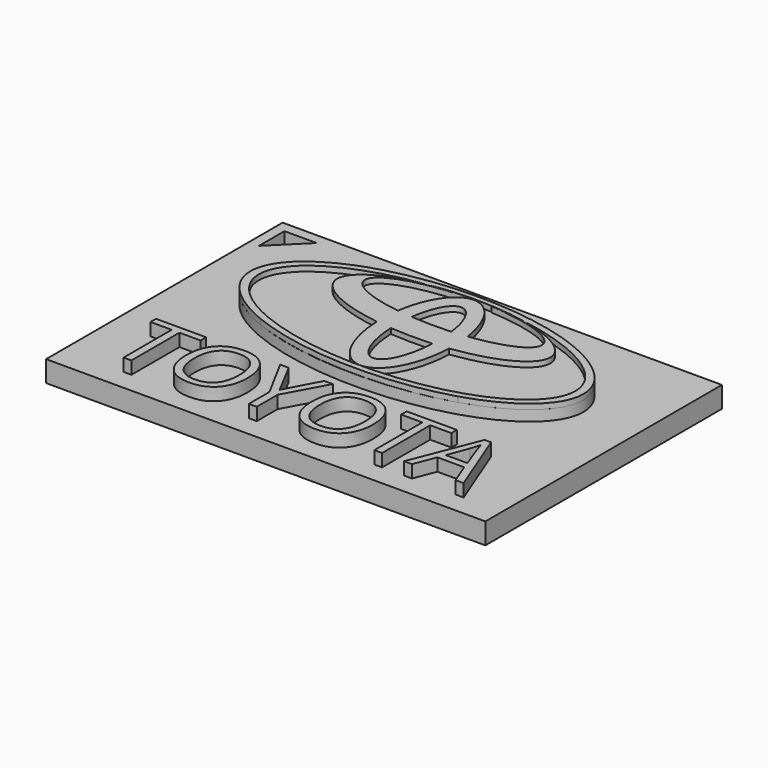
from build123d import *

# Parameters (mm, degrees)
F0_W         = 66.04
F0_H         = 44.45
F0_TEXT_SIZE = 14.1111111111
F1_DEPTH     = 3.175
F2_DEPTH     = 1.5875
F4_DEPTH     = 1.905
F6_DEPTH     = 0.79375


# Not quite as in the source:
# - a feature names something its author has since deleted; it is built from what else it names
# - Text() gives the source's letters only with a copy of the font that has no kerning and outlines rounded to 1/6400 em; it was checked with that copy


with BuildPart() as f1:
    # F0 (on Top) → F1 (new body)
    with BuildSketch(Plane.XY):
        with Locations((3.48807069, -6.6769314361)):
            Rectangle(F0_W, F0_H)
        Polygon((-19.2232334766, -16.7264181777), (-19.2232334766, -25.7597341499), (-20.3940147266, -25.7597341499), (-20.3940147266, -16.7264181777), (-23.5844487544, -16.7264181777), (-23.5844487544, -15.6857237332), (-16.0327994489, -15.6857237332), (-16.0327994489, -16.7264181777), align=None, mode=Mode.SUBTRACT)
        with BuildLine():
            add(Edge.make_bspline(
                [(-6.9906640322, -16.9050119277), (-5.7713758378, -18.2830501221), (-5.7713758378, -20.7083973443)],
                knots=[0, 0, 0, 1, 1, 1], degree=2))
            add(Edge.make_bspline(
                [(-5.7713758378, -20.7083973443), (-5.7713758378, -23.1271299832), (-6.9950737544, -24.5128851915)],
                knots=[0, 0, 0, 1, 1, 1], degree=2))
            add(Edge.make_bspline(
                [(-6.9950737544, -24.5128851915), (-8.2187716711, -25.8986403999), (-10.3949695878, -25.8986403999)],
                knots=[0, 0, 0, 1, 1, 1], degree=2))
            add(Edge.make_bspline(
                [(-10.3949695878, -25.8986403999), (-12.6196744489, -25.8986403999), (-13.8290407683, -24.5371386638)],
                knots=[0, 0, 0, 1, 1, 1], degree=2))
            add(Edge.make_bspline(
                [(-13.8290407683, -24.5371386638), (-15.0384070878, -23.1756369277), (-15.0384070878, -20.6951681777)],
                knots=[0, 0, 0, 1, 1, 1], degree=2))
            add(Edge.make_bspline(
                [(-15.0384070878, -20.6951681777), (-15.0384070878, -18.2345431777), (-13.8257334766, -16.8807584554)],
                knots=[0, 0, 0, 1, 1, 1], degree=2))
            add(Edge.make_bspline(
                [(-13.8257334766, -16.8807584554), (-12.6130598655, -15.5269737332), (-10.3817404211, -15.5269737332)],
                knots=[0, 0, 0, 1, 1, 1], degree=2))
            add(Edge.make_bspline(
                [(-10.3817404211, -15.5269737332), (-8.2099522266, -15.5269737332), (-6.9906640322, -16.9050119277)],
                knots=[0, 0, 0, 1, 1, 1], degree=2))
        make_face(mode=Mode.SUBTRACT)
        Polygon((-3.6304556989, -15.6857237332), (-0.9625737544, -20.7238313721), (1.7229470789, -15.6857237332), (2.9907422178, -15.6857237332), (-0.3716709766, -21.852720261), (-0.3716709766, -25.7597341499), (-1.5556813933, -25.7597341499), (-1.5556813933, -21.9078417888), (-4.9114800044, -15.6857237332), align=None, mode=Mode.SUBTRACT)
        with BuildLine():
            add(Edge.make_bspline(
                [(11.9005859678, -16.9050119277), (13.1198741622, -18.2830501221), (13.1198741622, -20.7083973443)],
                knots=[0, 0, 0, 1, 1, 1], degree=2))
            add(Edge.make_bspline(
                [(13.1198741622, -20.7083973443), (13.1198741622, -23.1271299832), (11.8961762456, -24.5128851915)],
                knots=[0, 0, 0, 1, 1, 1], degree=2))
            add(Edge.make_bspline(
                [(11.8961762456, -24.5128851915), (10.6724783289, -25.8986403999), (8.4962804122, -25.8986403999)],
                knots=[0, 0, 0, 1, 1, 1], degree=2))
            add(Edge.make_bspline(
                [(8.4962804122, -25.8986403999), (6.2715755511, -25.8986403999), (5.0622092317, -24.5371386638)],
                knots=[0, 0, 0, 1, 1, 1], degree=2))
            add(Edge.make_bspline(
                [(5.0622092317, -24.5371386638), (3.8528429122, -23.1756369277), (3.8528429122, -20.6951681777)],
                knots=[0, 0, 0, 1, 1, 1], degree=2))
            add(Edge.make_bspline(
                [(3.8528429122, -20.6951681777), (3.8528429122, -18.2345431777), (5.0655165234, -16.8807584554)],
                knots=[0, 0, 0, 1, 1, 1], degree=2))
            add(Edge.make_bspline(
                [(5.0655165234, -16.8807584554), (6.2781901345, -15.5269737332), (8.5095095789, -15.5269737332)],
                knots=[0, 0, 0, 1, 1, 1], degree=2))
            add(Edge.make_bspline(
                [(8.5095095789, -15.5269737332), (10.6812977734, -15.5269737332), (11.9005859678, -16.9050119277)],
                knots=[0, 0, 0, 1, 1, 1], degree=2))
        make_face(mode=Mode.SUBTRACT)
        Polygon((18.4644574956, -16.7264181777), (18.4644574956, -25.7597341499), (17.2936762456, -25.7597341499), (17.2936762456, -16.7264181777), (14.1032422178, -16.7264181777), (14.1032422178, -15.6857237332), (21.6548915234, -15.6857237332), (21.6548915234, -16.7264181777), align=None, mode=Mode.SUBTRACT)
        Polygon((30.71687069, -25.7597341499), (29.5041970789, -25.7597341499), (28.2496311067, -22.5560709554), (24.2125304122, -22.5560709554), (22.9733984678, -25.7597341499), (21.78718319, -25.7597341499), (25.7691623567, -15.6438313721), (26.7547352734, -15.6438313721), align=None, mode=Mode.SUBTRACT)
        with BuildLine():
            add(Edge.make_bspline(
                [(-21.91192931, 0), (-21.91192931, -20.151710611), (15.61657069, -10.0758553055), (53.14507069, 0), (15.61657069, 10.0758553055), (-21.91192931, 20.151710611), (-21.91192931, 0)],
                knots=[0, 0, 0, 2.0943951024, 2.0943951024, 4.1887902048, 4.1887902048, 6.2831853072, 6.2831853072, 6.2831853072], degree=2, weights=[1, 0.5, 1, 0.5, 1, 0.5, 1]))
        make_face(mode=Mode.SUBTRACT)
        Polygon((-28.00792931, 9.1980685639), (-28.00792931, 13.9852360981), (-23.18192931, 13.9852360981), align=None, mode=Mode.SUBTRACT)
        with BuildLine():
            add(Edge.make_bspline(
                [(-21.91192931, 0), (-21.91192931, -20.151710611), (15.61657069, -10.0758553055), (53.14507069, 0), (15.61657069, 10.0758553055), (-21.91192931, 20.151710611), (-21.91192931, 0)],
                knots=[0, 0, 0, 2.0943951024, 2.0943951024, 4.1887902048, 4.1887902048, 6.2831853072, 6.2831853072, 6.2831853072], degree=2, weights=[1, 0.5, 1, 0.5, 1, 0.5, 1]))
        make_face()
        with BuildLine():
            add(Edge.make_bspline(
                [(-12.9272525739, -17.6326160943), (-13.7992751433, -18.6909494277), (-13.7992751433, -20.7083973443)],
                knots=[0, 0, 0, 1, 1, 1], degree=2))
            add(Edge.make_bspline(
                [(-13.7992751433, -20.7083973443), (-13.7992751433, -22.7545084554), (-12.9272525739, -23.8128417888)],
                knots=[0, 0, 0, 1, 1, 1], degree=2))
            add(Edge.make_bspline(
                [(-12.9272525739, -23.8128417888), (-12.0552300044, -24.8711751221), (-10.3949695878, -24.8711751221)],
                knots=[0, 0, 0, 1, 1, 1], degree=2))
            add(Edge.make_bspline(
                [(-10.3949695878, -24.8711751221), (-8.7214800044, -24.8711751221), (-7.8670963239, -23.817251511)],
                knots=[0, 0, 0, 1, 1, 1], degree=2))
            add(Edge.make_bspline(
                [(-7.8670963239, -23.817251511), (-7.0127126433, -22.7633278999), (-7.0127126433, -20.7083973443)],
                knots=[0, 0, 0, 1, 1, 1], degree=2))
            add(Edge.make_bspline(
                [(-7.0127126433, -20.7083973443), (-7.0127126433, -18.6755153999), (-7.8637890322, -17.6248990804)],
                knots=[0, 0, 0, 1, 1, 1], degree=2))
            add(Edge.make_bspline(
                [(-7.8637890322, -17.6248990804), (-8.7148654211, -16.574282761), (-10.3817404211, -16.574282761)],
                knots=[0, 0, 0, 1, 1, 1], degree=2))
            add(Edge.make_bspline(
                [(-10.3817404211, -16.574282761), (-12.0552300044, -16.574282761), (-12.9272525739, -17.6326160943)],
                knots=[0, 0, 0, 1, 1, 1], degree=2))
        make_face()
        with BuildLine():
            add(Edge.make_bspline(
                [(5.9639974261, -17.6326160943), (5.0919748567, -18.6909494277), (5.0919748567, -20.7083973443)],
                knots=[0, 0, 0, 1, 1, 1], degree=2))
            add(Edge.make_bspline(
                [(5.0919748567, -20.7083973443), (5.0919748567, -22.7545084554), (5.9639974261, -23.8128417888)],
                knots=[0, 0, 0, 1, 1, 1], degree=2))
            add(Edge.make_bspline(
                [(5.9639974261, -23.8128417888), (6.8360199956, -24.8711751221), (8.4962804122, -24.8711751221)],
                knots=[0, 0, 0, 1, 1, 1], degree=2))
            add(Edge.make_bspline(
                [(8.4962804122, -24.8711751221), (10.1697699956, -24.8711751221), (11.0241536761, -23.817251511)],
                knots=[0, 0, 0, 1, 1, 1], degree=2))
            add(Edge.make_bspline(
                [(11.0241536761, -23.817251511), (11.8785373567, -22.7633278999), (11.8785373567, -20.7083973443)],
                knots=[0, 0, 0, 1, 1, 1], degree=2))
            add(Edge.make_bspline(
                [(11.8785373567, -20.7083973443), (11.8785373567, -18.6755153999), (11.0274609678, -17.6248990804)],
                knots=[0, 0, 0, 1, 1, 1], degree=2))
            add(Edge.make_bspline(
                [(11.0274609678, -17.6248990804), (10.1763845789, -16.574282761), (8.5095095789, -16.574282761)],
                knots=[0, 0, 0, 1, 1, 1], degree=2))
            add(Edge.make_bspline(
                [(8.5095095789, -16.574282761), (6.8360199956, -16.574282761), (5.9639974261, -17.6326160943)],
                knots=[0, 0, 0, 1, 1, 1], degree=2))
        make_face()
        with Locations((-23.7079209766, -25.7597341499)):
            Text('TOYOTA', F0_TEXT_SIZE, font='Open Sans', text_align=(TextAlign.LEFT, TextAlign.BOTTOM))
        with BuildLine():
            Line((24.6270443011, -21.5021473443), (27.8858290234, -21.5021473443))
            Line((27.8858290234, -21.5021473443), (26.7128429122, -18.380064011))
            add(Edge.make_bspline(
                [(26.7128429122, -18.380064011), (26.4857422178, -17.7869563721), (26.2454123567, -16.9270605388)],
                knots=[0, 0, 0, 1, 1, 1], degree=2))
            add(Edge.make_bspline(
                [(26.2454123567, -16.9270605388), (26.09327694, -17.5885188721), (25.8110547178, -18.380064011)],
                knots=[0, 0, 0, 1, 1, 1], degree=2))
            Line((25.8110547178, -18.380064011), (24.6270443011, -21.5021473443))
        make_face()
    extrude(amount=-F1_DEPTH)

    # F0 (on Top) → F2 (join)
    with BuildSketch(Plane.XY):
        with BuildLine():
            add(Edge.make_bspline(
                [(-21.91192931, 0), (-21.91192931, -20.151710611), (15.61657069, -10.0758553055), (53.14507069, 0), (15.61657069, 10.0758553055), (-21.91192931, 20.151710611), (-21.91192931, 0)],
                knots=[0, 0, 0, 2.0943951024, 2.0943951024, 4.1887902048, 4.1887902048, 6.2831853072, 6.2831853072, 6.2831853072], degree=2, weights=[1, 0.5, 1, 0.5, 1, 0.5, 1]))
        make_face()
    extrude(amount=F2_DEPTH)

    # F0 (on Top) → F4 (join)
    with BuildSketch(Plane.XY):
        with Locations((-23.7079209766, -25.7597341499)):
            Text('TOYOTA', F0_TEXT_SIZE, font='Open Sans', text_align=(TextAlign.LEFT, TextAlign.BOTTOM))
    extrude(amount=F4_DEPTH)


with BuildPart() as f6:
    # F5 (on face) → F6 (new body)
    with BuildSketch(Plane.XY.offset(1.5875)):
        with BuildLine():
            add(Edge.make_bspline(
                [(-21.91192931, 0), (-21.91192931, -5.3044246072), (-13.3008656787, -8.7831672199)],
                knots=[0, 0, 0, 0.872839559, 0.872839559, 0.872839559], degree=2, weights=[1, 0.7916249045, 0.7569305307]))
            add(Edge.make_bspline(
                [(-13.3008656787, -8.7831672199), (1.1436542695, -14.5267735488), (17.037322075, -9.6643393186)],
                knots=[0.8591280125, 0.8591280125, 0.8591280125, 2.1566382514, 2.1566382514, 2.1566382514], degree=2, weights=[1, 0.7968365663, 1]))
            add(Edge.make_bspline(
                [(17.037322075, -9.6643393186), (48.0416769439, 0), (17.037322075, 9.6643393186)],
                knots=[2.17380304, 2.17380304, 2.17380304, 4.1093822672, 4.1093822672, 4.1093822672], degree=2, weights=[0.9635230118, 0.5364769882, 0.9635230118]))
            add(Edge.make_bspline(
                [(17.037322075, 9.6643393186), (1.1436542695, 14.5267735488), (-13.3008656787, 8.7831672199)],
                knots=[4.1265470558, 4.1265470558, 4.1265470558, 5.4240572946, 5.4240572946, 5.4240572946], degree=2, weights=[1, 0.7968365663, 1]))
            add(Edge.make_bspline(
                [(-13.3008656787, 8.7831672199), (-21.91192931, 5.3044246072), (-21.91192931, 0)],
                knots=[5.4103457482, 5.4103457482, 5.4103457482, 6.2831853072, 6.2831853072, 6.2831853072], degree=2, weights=[0.7569305307, 0.7916249045, 1]))
        make_face()
        with BuildLine():
            add(Edge.make_bspline(
                [(-20.6518080086, 0), (-20.6518080086, -20.6316929025), (16.8327707214, -8.7419379974), (54.3173494513, 3.1478169077), (11.11367674, 10.0757122235)],
                knots=[0, 0, 0, 2.1849731253, 2.1849731253, 4.3699462507, 4.3699462507, 4.3699462507], degree=2, weights=[1, 0.460279286, 1, 0.460279286, 1]))
            add(Edge.make_bspline(
                [(-3.774671894, 10.2361811541), (-20.6518080086, 7.9332427254), (-20.6518080086, 0)],
                knots=[5.0069185112, 5.0069185112, 5.0069185112, 6.2831853072, 6.2831853072, 6.2831853072], degree=2, weights=[1, 0.8032090861, 1]))
            add(Edge.make_bspline(
                [(11.11367674, 10.0757122235), (3.782112381, 11.6187086605), (-3.774671894, 10.2361811541)],
                knots=[4.2000240201, 4.2000240201, 4.2000240201, 5.167159084, 5.167159084, 5.167159084], degree=2, weights=[1, 0.8853418698, 1]))
        make_face(mode=Mode.SUBTRACT)
    extrude(amount=F6_DEPTH)


with BuildPart() as f6b:
    # F5 (on face) → F6, piece 2 (new body)
    with BuildSketch(Plane.XY.offset(1.5875)):
        with BuildLine():
            add(Edge.make_bspline(
                [(8.5835805051, -0.8008267474), (41.9159642588, 3.5930821101), (11.11367674, 10.0757122235)],
                knots=[1.9095196694, 1.9095196694, 1.9095196694, 4.2000240201, 4.2000240201, 4.2000240201], degree=2, weights=[1, 0.4128164637, 1]))
            add(Edge.make_bspline(
                [(11.11367674, 10.0757122235), (8.535921546, 10.4890663902), (5.8168117785, 10.6282270657)],
                knots=[4.3699462507, 4.3699462507, 4.3699462507, 4.599099378, 4.599099378, 4.599099378], degree=2, weights=[1, 0.9934432832, 1]))
            add(Edge.make_bspline(
                [(16.5582895279, 6.6574071534), (16.5582895279, 9.9880882474), (5.8168117785, 10.6282270657)],
                knots=[0, 0, 0, 1.3773984076, 1.3773984076, 1.3773984076], degree=2, weights=[1, 0.7720733674, 1]))
            add(Edge.make_bspline(
                [(8.3886807252, 2.9240823869), (16.5582895279, 3.9630528795), (16.5582895279, 6.6574071534)],
                knots=[5.1082580599, 5.1082580599, 5.1082580599, 6.2831853072, 6.2831853072, 6.2831853072], degree=2, weights=[1, 0.8323491457, 1]))
            add(Edge.make_bspline(
                [(8.5835805051, -0.8008267474), (8.6570907099, 1.09550404), (8.3886807252, 2.9240823869)],
                knots=[1.4955016969, 1.4955016969, 1.4955016969, 1.8490384559, 1.8490384559, 1.8490384559], degree=2, weights=[1, 0.9844171101, 1]))
        make_face()
        with BuildLine():
            add(Edge.make_bspline(
                [(1.9135154193, 10.6828271367), (-0.991303057, 10.6159806065), (-3.774671894, 10.2361811541)],
                knots=[4.7635036137, 4.7635036137, 4.7635036137, 5.0069185112, 5.0069185112, 5.0069185112], degree=2, weights=[1, 0.9926027863, 1]))
            add(Edge.make_bspline(
                [(-3.774671894, 10.2361811541), (-12.7564836293, 8.592942267), (-12.7564836293, 4.8519810662)],
                knots=[5.167159084, 5.167159084, 5.167159084, 6.2831853072, 6.2831853072, 6.2831853072], degree=2, weights=[1, 0.8483088456, 1]))
            add(Edge.make_bspline(
                [(-12.7564836293, 4.8519810662), (-12.7564836293, 0.6882105932), (-2.327933538, -0.7646719816)],
                knots=[0, 0, 0, 1.2143625775, 1.2143625775, 1.2143625775], degree=2, weights=[1, 0.8212595076, 1]))
            add(Edge.make_bspline(
                [(-2.12662699, 2.9581827387), (-2.3981102976, 1.1317378567), (-2.327933538, -0.7646719816)],
                knots=[4.4308140133, 4.4308140133, 4.4308140133, 4.784278291, 4.784278291, 4.784278291], degree=2, weights=[1, 0.9844234823, 1]))
            add(Edge.make_bspline(
                [(1.9135154193, 10.6828271367), (-8.2629050259, 10.3673576061), (-9.8706586007, 7.2933757047), (-11.4784121756, 4.2193938033), (-2.12662699, 2.9581827387)],
                knots=[1.6723207858, 1.6723207858, 1.6723207858, 2.9837636011, 2.9837636011, 4.2952064164, 4.2952064164, 4.2952064164], degree=2, weights=[1, 0.7926082696, 1, 0.7926082696, 1]))
        make_face()
        with BuildLine():
            add(Edge.make_bspline(
                [(3.1285083387, -10.6459641829), (8.2019392463, -10.6459641829), (8.5835805051, -0.8008267474)],
                knots=[0, 0, 0, 1.4955016969, 1.4955016969, 1.4955016969], degree=2, weights=[1, 0.7332201258, 1]))
            add(Edge.make_bspline(
                [(6.2829505478, -1.0337540258), (7.4564868066, -0.9494013895), (8.5835805051, -0.8008267474)],
                knots=[1.7605860862, 1.7605860862, 1.7605860862, 1.9095196694, 1.9095196694, 1.9095196694], degree=2, weights=[1, 0.9972286295, 1]))
            add(Edge.make_bspline(
                [(3.1285083387, -8.2652829587), (5.9322779633, -8.2652829587), (6.2829505478, -1.0337540258)],
                knots=[0, 0, 0, 1.4453961023, 1.4453961023, 1.4453961023], degree=2, weights=[1, 0.7500239414, 1]))
            add(Edge.make_bspline(
                [(-0.0268950956, -1.0137348931), (0.3178334753, -8.2652829587), (3.1285083387, -8.2652829587)],
                knots=[4.8353483339, 4.8353483339, 4.8353483339, 6.2831853072, 6.2831853072, 6.2831853072], degree=2, weights=[1, 0.7492161739, 1]))
            add(Edge.make_bspline(
                [(-2.327933538, -0.7646719816), (-1.2023701135, -0.9214829929), (-0.0268950956, -1.0137348931)],
                knots=[1.2143625775, 1.2143625775, 1.2143625775, 1.3640485349, 1.3640485349, 1.3640485349], degree=2, weights=[1, 0.9972005714, 1]))
            add(Edge.make_bspline(
                [(-2.327933538, -0.7646719816), (-1.9622757287, -10.6459641829), (3.1285083387, -10.6459641829)],
                knots=[4.784278291, 4.784278291, 4.784278291, 6.2831853072, 6.2831853072, 6.2831853072], degree=2, weights=[1, 0.7320612697, 1]))
        make_face()
        with BuildLine():
            add(Edge.make_bspline(
                [(6.2829505478, -1.0337540258), (7.4564868066, -0.9494013895), (8.5835805051, -0.8008267474)],
                knots=[1.7605860862, 1.7605860862, 1.7605860862, 1.9095196694, 1.9095196694, 1.9095196694], degree=2, weights=[1, 0.9972286295, 1]))
            add(Edge.make_bspline(
                [(8.5835805051, -0.8008267474), (8.6570907099, 1.09550404), (8.3886807252, 2.9240823869)],
                knots=[1.4955016969, 1.4955016969, 1.4955016969, 1.8490384559, 1.8490384559, 1.8490384559], degree=2, weights=[1, 0.9844171101, 1]))
            add(Edge.make_bspline(
                [(6.1326102547, 2.7066205915), (7.2925690992, 2.7846843247), (8.3886807252, 2.9240823869)],
                knots=[4.9300474937, 4.9300474937, 4.9300474937, 5.1082580599, 5.1082580599, 5.1082580599], degree=2, weights=[1, 0.9960327502, 1]))
            add(Edge.make_bspline(
                [(6.2829505478, -1.0337540258), (6.375853883, 0.882087662), (6.1326102547, 2.7066205915)],
                knots=[1.4453961023, 1.4453961023, 1.4453961023, 1.9044195265, 1.9044195265, 1.9044195265], degree=2, weights=[1, 0.9737775976, 1]))
        make_face()
        with BuildLine():
            add(Edge.make_bspline(
                [(-0.0268950956, -1.0137348931), (3.1226531712, -1.2609131044), (6.2829505478, -1.0337540258)],
                knots=[1.3640485349, 1.3640485349, 1.3640485349, 1.7605860862, 1.7605860862, 1.7605860862], degree=2, weights=[1, 0.9804090502, 1]))
            add(Edge.make_bspline(
                [(6.2829505478, -1.0337540258), (6.375853883, 0.882087662), (6.1326102547, 2.7066205915)],
                knots=[1.4453961023, 1.4453961023, 1.4453961023, 1.9044195265, 1.9044195265, 1.9044195265], degree=2, weights=[1, 0.9737775976, 1]))
            add(Edge.make_bspline(
                [(0.1268880909, 2.7251639918), (3.1226854858, 2.5040565394), (6.1326102547, 2.7066205915)],
                knots=[4.4744376073, 4.4744376073, 4.4744376073, 4.9300474937, 4.9300474937, 4.9300474937], degree=2, weights=[1, 0.9741644725, 1]))
            add(Edge.make_bspline(
                [(0.1268880909, 2.7251639918), (-0.1179858584, 0.902407547), (-0.0268950956, -1.0137348931)],
                knots=[4.3763903496, 4.3763903496, 4.3763903496, 4.8353483339, 4.8353483339, 4.8353483339], degree=2, weights=[1, 0.9737850409, 1]))
        make_face()
        with BuildLine():
            add(Edge.make_bspline(
                [(6.1326102547, 2.7066205915), (7.2925690992, 2.7846843247), (8.3886807252, 2.9240823869)],
                knots=[4.9300474937, 4.9300474937, 4.9300474937, 5.1082580599, 5.1082580599, 5.1082580599], degree=2, weights=[1, 0.9960327502, 1]))
            add(Edge.make_bspline(
                [(8.3886807252, 2.9240823869), (3.1615062565, 38.5348964167), (-2.12662699, 2.9581827387)],
                knots=[1.8490384559, 1.8490384559, 1.8490384559, 4.4308140133, 4.4308140133, 4.4308140133], degree=2, weights=[1, 0.2762677571, 1]))
            add(Edge.make_bspline(
                [(-2.12662699, 2.9581827387), (-1.0342737928, 2.8108645623), (0.1268880909, 2.7251639918)],
                knots=[4.2952064164, 4.2952064164, 4.2952064164, 4.4744376073, 4.4744376073, 4.4744376073], degree=2, weights=[1, 0.9959872092, 1]))
            add(Edge.make_bspline(
                [(6.1326102547, 2.7066205915), (3.1400005468, 25.1537243314), (0.1268880909, 2.7251639918)],
                knots=[1.9044195265, 1.9044195265, 1.9044195265, 4.3763903496, 4.3763903496, 4.3763903496], degree=2, weights=[1, 0.3285905904, 1]))
        make_face()
        with BuildLine():
            add(Edge.make_bspline(
                [(-2.12662699, 2.9581827387), (-1.0342737928, 2.8108645623), (0.1268880909, 2.7251639918)],
                knots=[4.2952064164, 4.2952064164, 4.2952064164, 4.4744376073, 4.4744376073, 4.4744376073], degree=2, weights=[1, 0.9959872092, 1]))
            add(Edge.make_bspline(
                [(-2.12662699, 2.9581827387), (-2.3981102976, 1.1317378567), (-2.327933538, -0.7646719816)],
                knots=[4.4308140133, 4.4308140133, 4.4308140133, 4.784278291, 4.784278291, 4.784278291], degree=2, weights=[1, 0.9844234823, 1]))
            add(Edge.make_bspline(
                [(-2.327933538, -0.7646719816), (-1.2023701135, -0.9214829929), (-0.0268950956, -1.0137348931)],
                knots=[1.2143625775, 1.2143625775, 1.2143625775, 1.3640485349, 1.3640485349, 1.3640485349], degree=2, weights=[1, 0.9972005714, 1]))
            add(Edge.make_bspline(
                [(0.1268880909, 2.7251639918), (-0.1179858584, 0.902407547), (-0.0268950956, -1.0137348931)],
                knots=[4.3763903496, 4.3763903496, 4.3763903496, 4.8353483339, 4.8353483339, 4.8353483339], degree=2, weights=[1, 0.9737850409, 1]))
        make_face()
    extrude(amount=F6_DEPTH)


solid = Compound([f1.part, f6.part, f6b.part])
